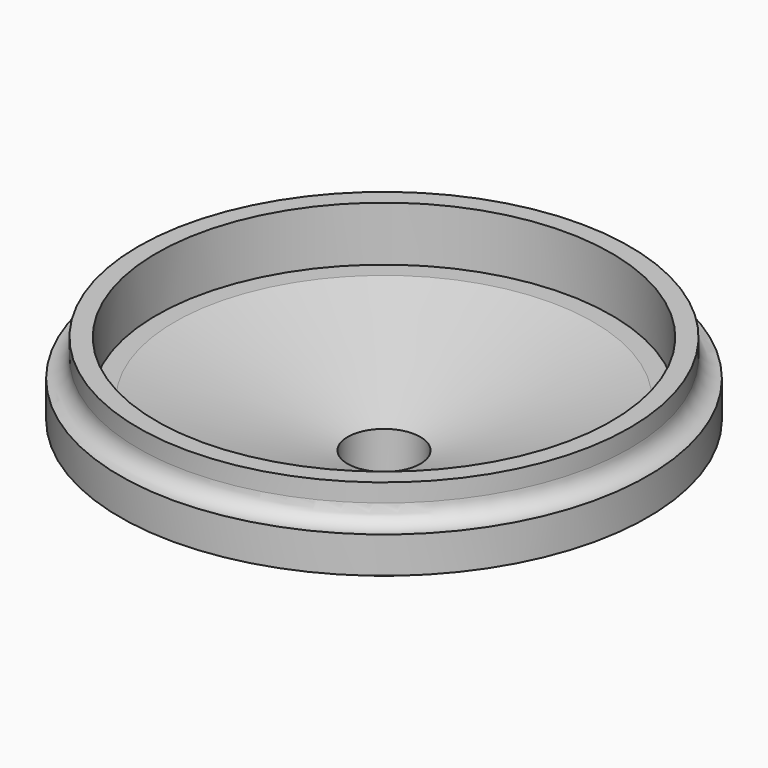
from build123d import *

# Parameters (mm, degrees)
F0_W     = 2
F0_H     = 4
F4_R     = 5
F5_R     = 4
F6_DEPTH = 25
F7_R     = 1.99999


# Not quite as in the source:
# - a fillet or chamfer is up to 0.001 mm smaller than in the source, because OpenCascade refuses the exact size
# - a feature names something its author has since deleted; it is built from what else it names


with BuildPart() as f1:
    # F0 (on Right) → F1 (revolve)
    with BuildSketch(Plane.YZ):
        with Locations((-26, 6)):
            Rectangle(F0_W, F0_H)
        Polygon((-29, 0), (-25, 0), (-25, 2), (-25, 4), (-27, 4), (-29, 4), align=None)
        Polygon((-25, 2), (-25, 0), (-23.256576216, 0), (0, -6.0669329259), (0, -4), (-23, 2), align=None)
    revolve(axis=Axis((0, 0, 1), (0, 0, 1)))

    # F2 (on Right) → F3 (revolve)
    with BuildSketch(Plane.YZ):
        Polygon((-10, -8), (-6, -8), (-6, -12), (0, -12), (0, -4), (-10, -1.3913043478), align=None)
    revolve(axis=Axis((0, 0, -8), (0, 0, 1)))

    # F4
    f4_edges = [f1.edges().sort_by_distance(p)[0] for p in [
        (0, 10, -3.458237),
    ]]
    fillet(f4_edges, radius=F4_R)

    # F5 (on Top) → F6 (cut)
    with BuildSketch(Plane.XY):
        Circle(F5_R)
    extrude(amount=-F6_DEPTH, mode=Mode.SUBTRACT)

    # F7 (radius 2 in the source; OpenCascade refuses exactly that, so slightly less here)
    f7_edges = [f1.edges().sort_by_distance(p)[0] for p in [
        (0, 27, 4),
    ]]
    fillet(f7_edges, radius=F7_R)


solid = f1.part
